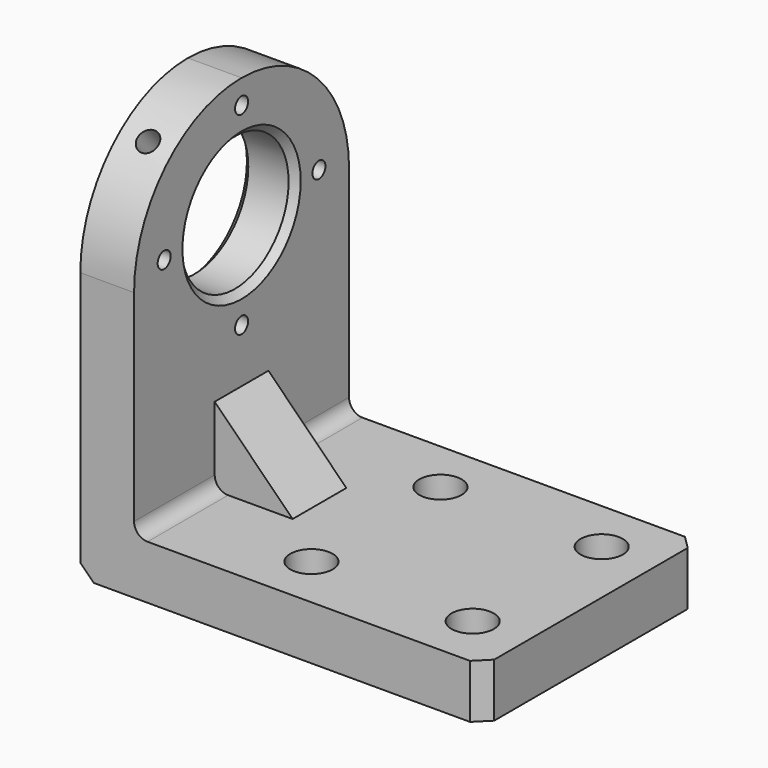
from build123d import *

# Parameters (mm, degrees)
F0_W      = 300
F0_H      = 200
F1_DEPTH  = 300
F2_W      = 260
F2_H      = 260
F3_DEPTH  = 421.64
F4_SIZE   = 10
F5_R      = 10
F6_SIZE   = 10
F7_R      = 8.75
F8_DEPTH  = 79.502
F7_R_2    = 15.75
F9_DEPTH  = 20
F10_R     = 99.99999
F11_R     = 50
F12_DEPTH = 145.034
F13_D     = 12.1
F14_SIZE  = 5
F16_DEPTH = 25
F20_D     = 15.5
F20_DEPTH = 44.0944
F20_START = 0.8055971
F20_TIP   = 4.6566697975


# Not quite as in the source:
# - a fillet or chamfer is up to 0.001 mm smaller than in the source, because OpenCascade refuses the exact size


with BuildPart() as f1:
    # F0 (on Top) → F1 (new body)
    with BuildSketch(Plane.XY):
        Rectangle(F0_W, F0_H)
    extrude(amount=F1_DEPTH)

    # F2 (on face) → F3 (cut)
    with BuildSketch(Plane.XZ.offset(100)):
        with Locations((20, 170)):
            Rectangle(F2_W, F2_H)
    extrude(amount=-F3_DEPTH, mode=Mode.SUBTRACT)

    # F4
    f4_edges = [f1.edges().sort_by_distance(p)[0] for p in [
        (150, -100, 20),
        (150, 100, 20),
    ]]
    chamfer(f4_edges, length=F4_SIZE)

    # F5
    f5_edges = [f1.edges().sort_by_distance(p)[0] for p in [
        (-110, 0, 40),
    ]]
    fillet(f5_edges, radius=F5_R)

    # F6
    f6_edges = [f1.edges().sort_by_distance(p)[0] for p in [
        (-150, 0, 0),
    ]]
    chamfer(f6_edges, length=F6_SIZE)

    # F7 (on face) → F8 (cut)
    with BuildSketch(Plane.XY.offset(40)):
        with Locations((110, -60)):
            Circle(F7_R)
        with Locations((110, 60)):
            Circle(F7_R)
        with Locations((-10, 60)):
            Circle(F7_R)
        with Locations((-10, -60)):
            Circle(F7_R)
    extrude(amount=-F8_DEPTH, mode=Mode.SUBTRACT)

    # F7 (on face) → F9 (cut)
    with BuildSketch(Plane.XY.offset(40)):
        with Locations((-10, 60)):
            Circle(F7_R_2)
        with Locations((-10, 60)):
            Circle(F7_R, mode=Mode.SUBTRACT)
        with Locations((-10, -60)):
            Circle(F7_R_2)
        with Locations((-10, -60)):
            Circle(F7_R, mode=Mode.SUBTRACT)
        with Locations((110, -60)):
            Circle(F7_R_2)
        with Locations((110, -60)):
            Circle(F7_R, mode=Mode.SUBTRACT)
        with Locations((110, 60)):
            Circle(F7_R_2)
        with Locations((110, 60)):
            Circle(F7_R, mode=Mode.SUBTRACT)
    extrude(amount=-F9_DEPTH, mode=Mode.SUBTRACT)

    # F10 (radius 100 in the source; OpenCascade refuses exactly that, so slightly less here)
    f10_edges = [f1.edges().sort_by_distance(p)[0] for p in [
        (-130, -100, 300),
        (-130, 100, 300),
    ]]
    fillet(f10_edges, radius=F10_R)

    # F11 (on face) → F12 (cut)
    with BuildSketch(Plane.YZ.offset(-110)):
        with Locations((0, 210.0496292114)):
            Circle(F11_R)
    extrude(amount=-F12_DEPTH, mode=Mode.SUBTRACT)

    # F13 (through all)
    with Locations(Plane.YZ.offset(-110)):
        with Locations((-72, 210.0496292114), (0, 282.0496292114), (71.9983499009, 210.5370833633), (0, 138.0496292114)):
            Hole(F13_D / 2)

    # F14
    f14_edges = [f1.edges().sort_by_distance(p)[0] for p in [
        (-150, -50, 210.049629),
        (-110, -50, 210.049629),
    ]]
    chamfer(f14_edges, length=F14_SIZE)

    # F15 (on Front) → F16 (join, symmetric)
    with BuildSketch(Plane.XZ):
        Polygon((-51.5841689292, 39.5744924862), (-111.5841689292, 99.5744924862), (-111.5841689292, 39.5744924862), align=None)
    extrude(amount=F16_DEPTH, both=True)

    # F20
    # its depths count from where the whole tool has entered the part; down to there all is cleared
    with Locations(Plane(origin=(0, -166.0770217272, 185.5655664485), x_dir=(1, 0, 0), z_dir=(0, -0.6668944822, 0.7451521654)).offset(-F20_START)):
        with Locations((-129.2792707682, 138.2966190577)):
            Hole(F20_D / 2, depth=F20_DEPTH)
            with Locations((0, 0, -(F20_DEPTH + F20_TIP / 2))):  # 118° drill point
                Cone(0, F20_D / 2, F20_TIP, mode=Mode.SUBTRACT)


solid = f1.part
